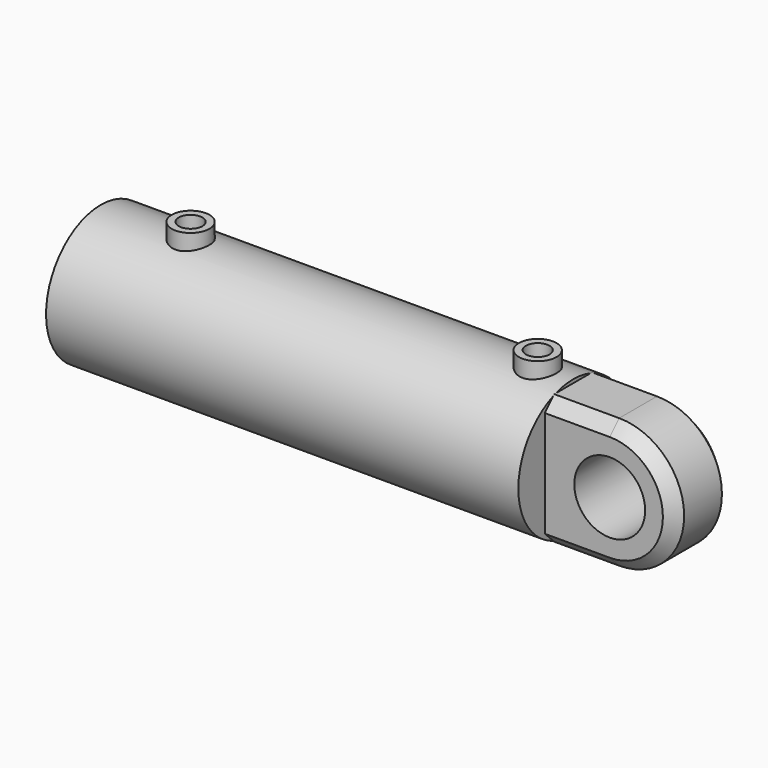
from build123d import *

# Parameters (mm, degrees)
F4_DEPTH    = 15
F5_T1_DEPTH = 27.5
F5_T4_ANGLE = 180
F5_T6_ANGLE = 180
F7_R        = 8
F7_R_2      = 5
F9_D        = 6
F9_DEPTH    = 20
F9_START    = 6.1555899
F9_TIP      = 1.8025818571
F10_D       = 6
F10_DEPTH   = 20
F10_START   = 6.1555899
F10_TIP     = 1.8025818571


# Not quite as in the source:
# - a fillet or chamfer that OpenCascade refuses, or shapes differently, is made with other operations: its cross-section is extruded or revolved along the edge and cut away or added


with BuildPart() as f3:
    # F2 (on Front) → F3 (revolve)
    with BuildSketch(Plane.XZ):
        Polygon((105.0486442498, 29), (98.7043133404, 29), (98.7043133404, 25.5), (105.7043133404, 25.5), (107.0780520501, 25), (250.7043133404, 25), (250.7043133404, 0), (260.7043133404, 0), (260.7043133404, 27.5), (260.7043133404, 29), align=None)
        Polygon((92.3599824309, 29), (60.7043133404, 29), (60.7043133404, 26.6542383736), (79.2043133404, 26.6542383736), (81.2035128474, 25.5), (98.7043133404, 25.5), (98.7043133404, 29), align=None)
    revolve(axis=Axis((125.4885941744, 0, 0), (1, 0, 0)))

    # F2 (on Front) → F4 (join, symmetric)
    with BuildSketch(Plane.XZ):
        with BuildLine():
            Line((288.2043133404, 27.5), (260.7043133404, 27.5))
            Line((260.7043133404, 27.5), (260.7043133404, 0))
            Line((260.7043133404, 0), (260.7043133404, -27.5))
            Line((260.7043133404, -27.5), (288.2043133404, -27.5))
            ThreePointArc((288.2043133404, -27.5), (315.7043133404, 0), (288.2043133404, 27.5))
        make_face()
        with BuildLine():
            ThreePointArc((303.2043133404, 0), (288.2043133404, -15), (273.2043133404, 0))
            ThreePointArc((273.2043133404, 0), (288.2043133404, 15), (303.2043133404, 0))
        make_face(mode=Mode.SUBTRACT)
    extrude(amount=F4_DEPTH, both=True)

    # F5: chamfer of 5 on 6 edges, made by hand

    # F5_s2 → F5_t1 (cut)
    with BuildSketch(Plane.YZ.offset(260.7043133404)):
        Polygon((-10, 27.5), (-15, 22.5), (-15, 27.5), align=None)
        Polygon((10, 27.5), (15, 22.5), (15, 27.5), align=None)
        Polygon((15, -22.5), (10, -27.5), (15, -27.5), align=None)
        Polygon((-10, -27.5), (-15, -22.5), (-15, -27.5), align=None)
    extrude(amount=F5_T1_DEPTH, mode=Mode.SUBTRACT)

    # F5_s3 → F5_t4 (revolve, cut)
    with BuildSketch(Plane.YZ.offset(288.2043133404)):
        Polygon((15, -22.5), (10, -27.5), (15, -27.5), align=None)
    revolve(axis=Axis((288.2043133404, 15, 0), (0, -1, 0)), revolution_arc=F5_T4_ANGLE, mode=Mode.SUBTRACT)

    # F5_s5 → F5_t6 (revolve, cut)
    with BuildSketch(Plane.YZ.offset(288.2043133404)):
        Polygon((-15, -22.5), (-10, -27.5), (-15, -27.5), align=None)
    revolve(axis=Axis((288.2043133404, -15, 0), (0, -1, 0)), revolution_arc=F5_T6_ANGLE, mode=Mode.SUBTRACT)

    # F7 (on offset) → F8 (join, up to the next surface of F3)
    with BuildSketch(Plane.XY.offset(35)):
        with Locations((98.7043133404, 0)):
            Circle(F7_R)
        with Locations((98.7043133404, 0)):
            Circle(F7_R_2, mode=Mode.SUBTRACT)
        with Locations((245.7043133404, 0)):
            Circle(F7_R)
        with Locations((245.7043133404, 0)):
            Circle(F7_R_2, mode=Mode.SUBTRACT)
    extrude(until=Until.NEXT, dir=(0, 0, -1))

    # F9
    # its depths count from where the whole tool has entered the part; down to there all is cleared
    with Locations(Plane.XY.offset(35).offset(-F9_START)):
        with Locations((98.7043133404, 0)):
            Hole(F9_D / 2, depth=F9_DEPTH)
            with Locations((0, 0, -(F9_DEPTH + F9_TIP / 2))):  # 118° drill point
                Cone(0, F9_D / 2, F9_TIP, mode=Mode.SUBTRACT)

    # F10
    # its depths count from where the whole tool has entered the part; down to there all is cleared
    with Locations(Plane.XY.offset(35).offset(-F10_START)):
        with Locations((245.7043133404, 0)):
            Hole(F10_D / 2, depth=F10_DEPTH)
            with Locations((0, 0, -(F10_DEPTH + F10_TIP / 2))):  # 118° drill point
                Cone(0, F10_D / 2, F10_TIP, mode=Mode.SUBTRACT)


solid = f3.part
